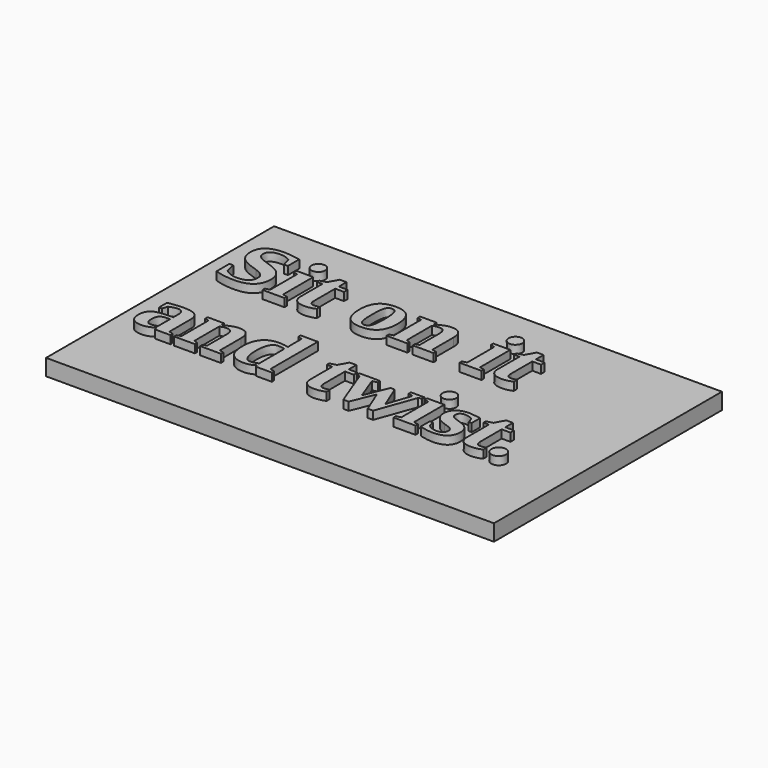
from build123d import *

# Parameters (mm, degrees)
F0_W         = 139.7
F0_H         = 88.9
F2_DEPTH     = 5.08
F1_TEXT_SIZE = 28.3650717595
F3_DEPTH     = 7.62


# Not quite as in the source:
# - Text() gives the source's letters only with a copy of the font that has no kerning and outlines rounded to 1/6400 em; it was checked with that copy


with BuildPart() as f2:
    # F0 (on Top) → F2 (new body)
    with BuildSketch(Plane.XY):
        Rectangle(F0_W, F0_H)
    extrude(amount=F2_DEPTH)

    # F1 (on face) → F3 (join)
    with BuildSketch(Plane.XY):
        with Locations((-64.4197203219, 12.6481400803)):
            Text('Sit on it', F1_TEXT_SIZE, font='Tinos', font_style=FontStyle.BOLD, text_align=(TextAlign.LEFT, TextAlign.BOTTOM))
        with Locations((-64.4197203219, -19.9716924431)):
            Text('and twist.', F1_TEXT_SIZE, font='Tinos', font_style=FontStyle.BOLD, text_align=(TextAlign.LEFT, TextAlign.BOTTOM))
    extrude(amount=F3_DEPTH)


solid = f2.part
